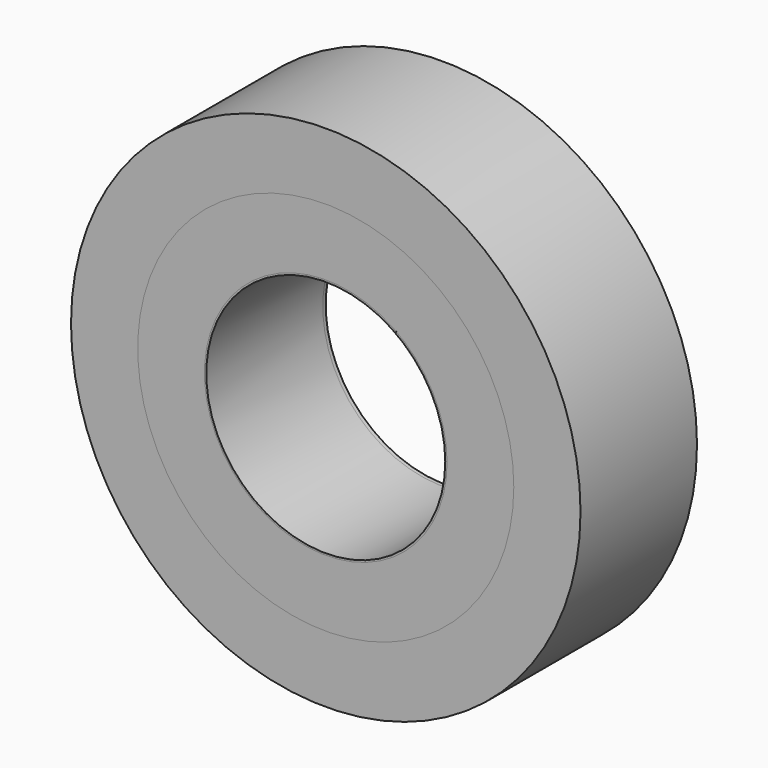
from build123d import *

# Parameters (mm, degrees)
F0_R     = 21
F0_R_2   = 15.5
F1_DEPTH = 12
F0_R_3   = 10
F2_DEPTH = 12
F3_R     = 10
F3_R_2   = 9.85
F4_DEPTH = 12
F3_R_3   = 11.5
F5_DEPTH = 0.3
F6_DEPTH = 25


with BuildPart() as f1:
    # F0 (on Front) → F1 (new body)
    with BuildSketch(Plane.XZ):
        Circle(F0_R)
        Circle(F0_R_2, mode=Mode.SUBTRACT)
    extrude(amount=F1_DEPTH)


with BuildPart() as f2:
    # F0 (on Front) → F2 (new body)
    with BuildSketch(Plane.XZ):
        Circle(F0_R_2)
        Circle(F0_R_3, mode=Mode.SUBTRACT)
    extrude(amount=F2_DEPTH)


with BuildPart() as f4:
    # F3 (on Front) → F4 (new body)
    with BuildSketch(Plane.XZ):
        Circle(F3_R)
        Circle(F3_R_2, mode=Mode.SUBTRACT)
    extrude(amount=F4_DEPTH)

    # F3 (on Front) → F5 (join)
    with BuildSketch(Plane.XZ):
        Circle(F3_R_3)
        Circle(F3_R, mode=Mode.SUBTRACT)
        Circle(F3_R)
        Circle(F3_R_2, mode=Mode.SUBTRACT)
        Circle(F3_R_2)
    extrude(amount=-F5_DEPTH)

    # F3 (on Front) → F6 (cut)
    with BuildSketch(Plane.XZ):
        Circle(F3_R_2)
    extrude(amount=-F6_DEPTH, mode=Mode.SUBTRACT)


solid = Compound([f1.part, f2.part, f4.part])
